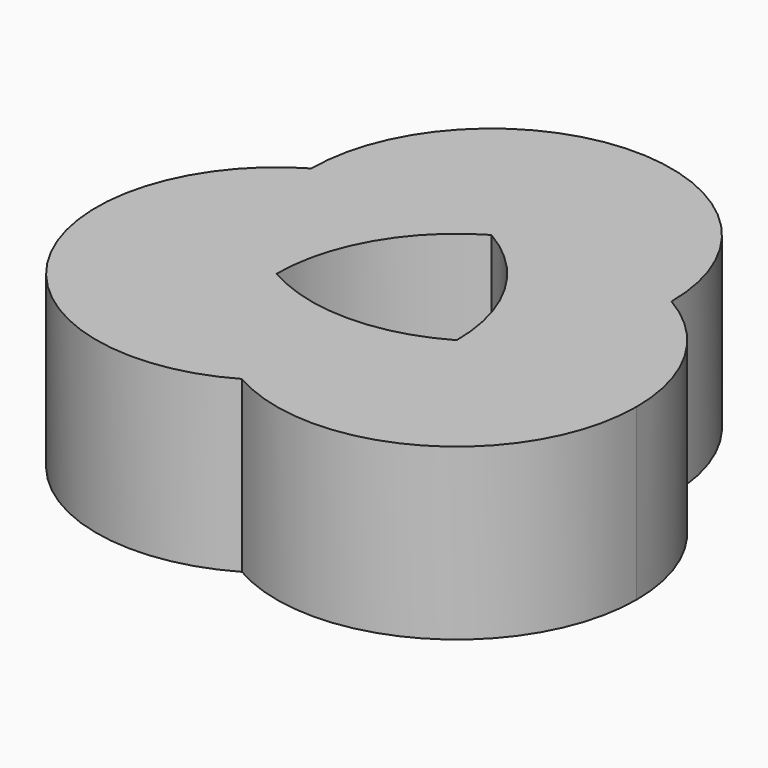
from build123d import *

# Parameters (mm, degrees)
F1_DEPTH = 25


with BuildPart() as f1:
    # F0 (on Top) → F1 (new body)
    with BuildSketch(Plane.XY):
        with BuildLine():
            ThreePointArc((-13.25, -22.9496732003), (13.25, -22.9496732003), (26.5, 0))
            ThreePointArc((26.5, 0), (22.9496732003, 13.25), (13.25, 22.9496732003))
            ThreePointArc((13.25, 22.9496732003), (9.6996732003, 9.6996732003), (0, 0))
            ThreePointArc((0, 0), (-3.5503267997, -13.25), (-13.25, -22.9496732003))
        make_face()
        with BuildLine():
            ThreePointArc((0, 0), (9.6996732003, 9.6996732003), (13.25, 22.9496732003))
            ThreePointArc((13.25, 22.9496732003), (0, 26.5), (-13.25, 22.9496732003))
            ThreePointArc((-13.25, 22.9496732003), (-3.5503267997, 13.25), (0, 0))
        make_face()
        with BuildLine():
            ThreePointArc((-13.25, 22.9496732003), (0, 26.5), (13.25, 22.9496732003))
            ThreePointArc((13.25, 22.9496732003), (-13.25, 49.4496732003), (-39.75, 22.9496732003))
            ThreePointArc((-39.75, 22.9496732003), (-26.5, 26.5), (-13.25, 22.9496732003))
        make_face()
        with BuildLine():
            ThreePointArc((-39.75, 22.9496732003), (-49.4496732003, -13.25), (-13.25, -22.9496732003))
            ThreePointArc((-13.25, -22.9496732003), (-22.9496732003, -13.25), (-26.5, 0))
            ThreePointArc((-26.5, 0), (-36.1996732003, 9.6996732003), (-39.75, 22.9496732003))
        make_face()
        with BuildLine():
            ThreePointArc((-26.5, 0), (-22.9496732003, -13.25), (-13.25, -22.9496732003))
            ThreePointArc((-13.25, -22.9496732003), (-3.5503267997, -13.25), (0, 0))
            ThreePointArc((0, 0), (-13.25, -3.5503267997), (-26.5, 0))
        make_face()
        with BuildLine():
            ThreePointArc((-26.5, 0), (-22.9496732003, 13.25), (-13.25, 22.9496732003))
            ThreePointArc((-13.25, 22.9496732003), (-26.5, 26.5), (-39.75, 22.9496732003))
            ThreePointArc((-39.75, 22.9496732003), (-36.1996732003, 9.6996732003), (-26.5, 0))
        make_face()
    extrude(amount=F1_DEPTH)


solid = f1.part
